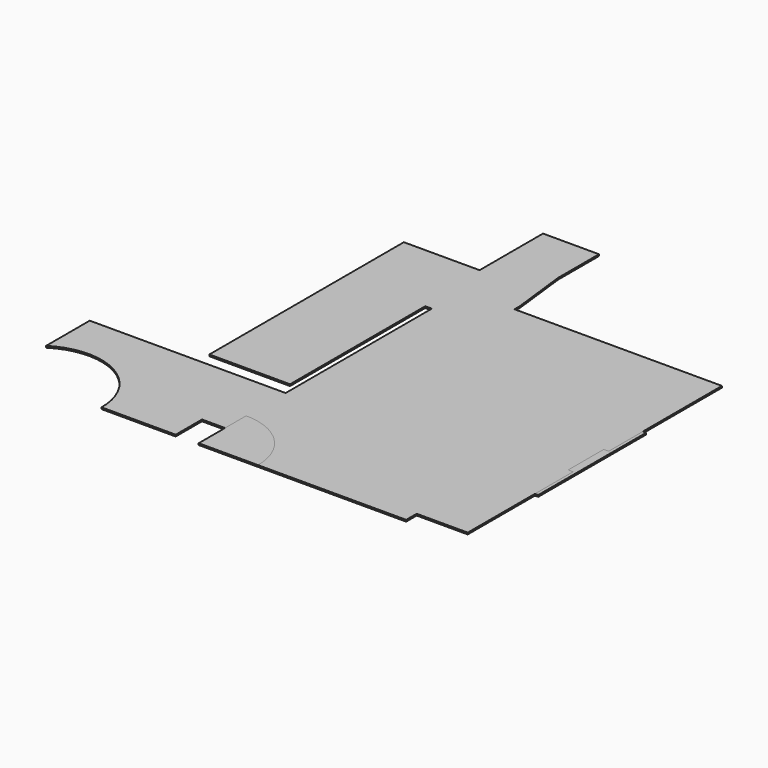
from build123d import *

# Parameters (mm, degrees)
F1_DEPTH = 25.4
F0_W     = 76.2
F0_H     = 685.8
F2_DEPTH = 25.4
F3_DEPTH = 25.4


# Not quite as in the source:
# - a feature names something its author has since deleted; it is built from what else it names


with BuildPart() as f1:
    # F0 (on Top) → F1 (new body)
    with BuildSketch(Plane.XY):
        with BuildLine():
            Line((914.4, 0), (3200.4, 0))
            Line((3200.4, 0), (3200.4, 203.2))
            Line((3200.4, 203.2), (3987.8, 203.2))
            Line((3987.8, 203.2), (3987.8, 1498.6))
            Line((3987.8, 1498.6), (3987.8, 2235.2))
            Line((3987.8, 2235.2), (3911.6, 2235.2))
            Line((3911.6, 2235.2), (3911.6, 2921))
            Line((3911.6, 2921), (3987.8, 2921))
            Line((3987.8, 2921), (3987.8, 3581.4))
            Line((3987.8, 3581.4), (3987.8, 5105.4))
            Line((3987.8, 5105.4), (787.4, 5105.4))
            Line((787.4, 5105.4), (787.4, 5207))
            Line((787.4, 5207), (701.3347370419, 5938.5547351442))
            Line((701.3347370419, 5938.5547351442), (685.8, 6070.6))
            Line((685.8, 6070.6), (685.8, 6862.3206634521))
            Line((685.8, 6862.3206634521), (-177.8, 6862.3206634521))
            Line((-177.8, 6862.3206634521), (-177.8, 6477))
            Line((-177.8, 6477), (-177.8, 5740.4))
            Line((-177.8, 5740.4), (-177.8, 5638.8))
            Line((-177.8, 5638.8), (-1346.2, 5638.8))
            Line((-1346.2, 5638.8), (-1346.2, 1888.175368309))
            Line((-1346.2, 1888.175368309), (-101.6, 1888.175368309))
            Line((-101.6, 1888.175368309), (-101.6, 4495.8))
            Line((-101.6, 4495.8), (0, 4495.8))
            Line((0, 4495.8), (0, 1676.4))
            Line((0, 1676.4), (-3022.6, 1676.4))
            Line((-3022.6, 1676.4), (-3022.6, 834.7291776379))
            ThreePointArc((-3022.6, 834.7291776379), (-2013.331152522, 868.8136739255), (-1498.6, 0))
            Line((-1498.6, 0), (-355.6, 0))
            Line((-355.6, 0), (-355.6, 508))
            Line((-355.6, 508), (0, 508))
            Line((0, 508), (0, 914.4))
            ThreePointArc((0, 914.4), (646.578440717, 646.578440717), (914.4, 0))
        make_face()
    extrude(amount=F1_DEPTH)


with BuildPart() as f2:
    # F0 (on Top) → F2 (new body)
    with BuildSketch(Plane.XY):
        with Locations((3949.7, 2578.1)):
            Rectangle(F0_W, F0_H)
        Polygon((3987.8, 2235.2), (3987.8, 1498.6), (4038.6, 1498.6), (4038.6, 3581.4), (3987.8, 3581.4), (3987.8, 2921), align=None)
    extrude(amount=F2_DEPTH)


with BuildPart() as f3:
    # F0 (on Top) → F3 (new body)
    with BuildSketch(Plane.XY):
        with BuildLine():
            Line((0, 0), (914.4, 0))
            ThreePointArc((914.4, 0), (646.578440717, 646.578440717), (0, 914.4))
            Line((0, 914.4), (0, 508))
            Line((0, 508), (0, 0))
        make_face()
    extrude(amount=F3_DEPTH)


solid = Compound([f1.part, f2.part, f3.part])
